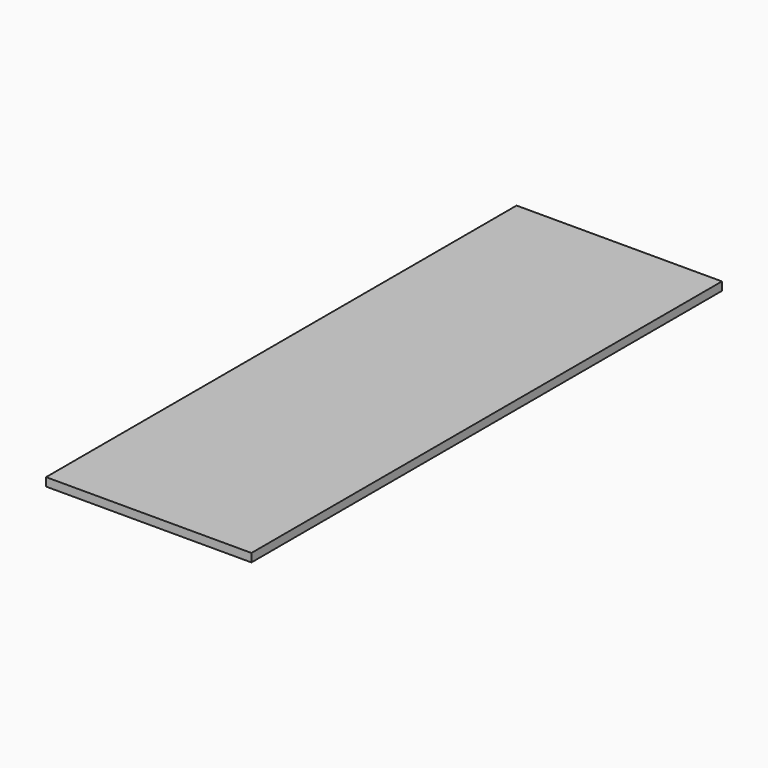
from build123d import *

# Parameters (mm, degrees)
F0_W     = 81.0896456242
F0_H     = 232.2407066822
F1_DEPTH = 3.302


with BuildPart() as f1:
    # F0 (on Top) → F1 (new body)
    with BuildSketch(Plane.XY):
        with Locations((260.1173371077, -116.1203533411)):
            Rectangle(F0_W, F0_H)
    extrude(amount=F1_DEPTH)


solid = f1.part
